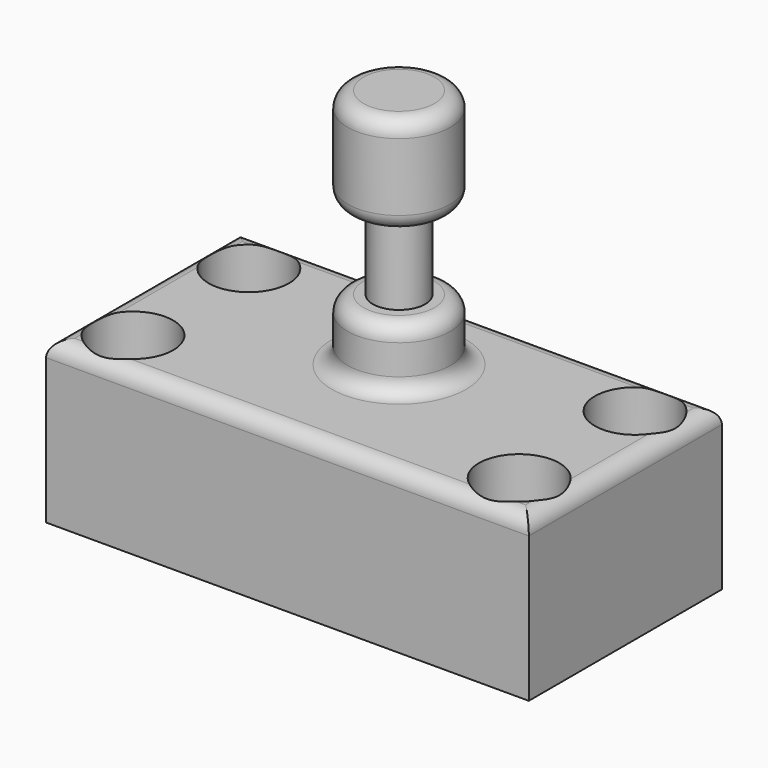
from build123d import *

# Parameters (mm, degrees)
F0_W        = 76.2
F0_H        = 38.1
F1_DEPTH    = 25.4
F2_R        = 6.35
F3_DEPTH    = 25.4
F4_R        = 8.1070086834
F5_DEPTH    = 38.1
F6_W        = 12.6953125
F6_H        = 12.6953087747
F8_T3_DEPTH = 50.8048285845
F8_T5_DEPTH = 88.9048285845


# Not quite as in the source:
# - a fillet or chamfer that OpenCascade refuses, or shapes differently, is made with other operations: its cross-section is extruded or revolved along the edge and cut away or added


with BuildPart() as f1:
    # F0 (on Top) → F1 (new body)
    with BuildSketch(Plane.XY):
        with Locations((-0.0034216791, -2.9583363167)):
            Rectangle(F0_W, F0_H)
    extrude(amount=F1_DEPTH)

    # F2 (on Top) → F3 (cut)
    with BuildSketch(Plane.XY):
        with Locations((-30.4834216791, 8.4716636833)):
            Circle(F2_R)
        with Locations((30.4765783209, 8.4716636833)):
            Circle(F2_R)
        with Locations((-30.4834216791, -14.3883363167)):
            Circle(F2_R)
        with Locations((30.4765783209, -14.3883363167)):
            Circle(F2_R)
    extrude(amount=F3_DEPTH, mode=Mode.SUBTRACT)

    # F4 (on face) → F5 (join)
    with BuildSketch(Plane.XY.offset(25.4)):
        Circle(F4_R)
    extrude(amount=F5_DEPTH)

    # F6 (on Front) → F7 (revolve, cut)
    with BuildSketch(Plane.XZ):
        with Locations((-10.4810148478, 41.481198743)):
            Rectangle(F6_W, F6_H)
    revolve(axis=Axis((0, 0, 25.4), (0, 0, -1)), mode=Mode.SUBTRACT)

    # F8: fillet of radius 2.54 on 8 edges, made by hand

    # F8_s1 → F8_t2 (revolve)
    with BuildSketch(Plane.XZ):
        with BuildLine():
            ThreePointArc((10.6479743688, 25.3996), (8.8509574592, 26.1439487758), (8.1066086834, 27.9409656854))
            Line((8.1066086834, 27.9409656854), (7.8524721149, 27.9409656854))
            ThreePointArc((7.8524721149, 27.9409656854), (7.8528721149, 26.6704828427), (7.8528721149, 25.4))
            Line((7.8528721149, 25.4), (8.1070086834, 25.1458634315))
            ThreePointArc((8.1070086834, 25.1458634315), (9.3774915261, 25.1458634315), (10.6479743688, 25.1454634315))
            Line((10.6479743688, 25.1454634315), (10.6479743688, 25.3996))
        make_face()
    revolve(axis=Axis((0, 0, 25.4), (0, 0, 1)))

    # F8_s4 → F8_t3 (cut)
    with BuildSketch(Plane.XZ.offset(-22.4440779756)):
        with BuildLine():
            ThreePointArc((-38.1038216791, 22.8590343146), (-37.3594729034, 24.6560512242), (-35.5624559937, 25.4004))
            Line((-35.5624559937, 25.4004), (-35.5624559937, 25.6545365685))
            ThreePointArc((-35.5624559937, 25.6545365685), (-36.8329388364, 25.6541365685), (-38.1034216791, 25.6541365685))
            Line((-38.1034216791, 25.6541365685), (-38.3575582477, 25.4))
            ThreePointArc((-38.3575582477, 25.4), (-38.3575582477, 24.1295171573), (-38.3579582477, 22.8590343146))
            Line((-38.3579582477, 22.8590343146), (-38.1038216791, 22.8590343146))
        make_face()
        with BuildLine():
            ThreePointArc((38.0969783209, 22.8590343146), (37.3526295451, 24.6560512242), (35.5556126354, 25.4004))
            Line((35.5556126354, 25.4004), (35.5556126354, 25.6545365685))
            ThreePointArc((35.5556126354, 25.6545365685), (36.8260954781, 25.6541365685), (38.0965783209, 25.6541365685))
            Line((38.0965783209, 25.6541365685), (38.3507148894, 25.4))
            ThreePointArc((38.3507148894, 25.4), (38.3507148894, 24.1295171573), (38.3511148894, 22.8590343146))
            Line((38.3511148894, 22.8590343146), (38.0969783209, 22.8590343146))
        make_face()
    extrude(amount=F8_T3_DEPTH, mode=Mode.SUBTRACT)

    # F8_s6 → F8_t5 (cut)
    with BuildSketch(Plane.YZ.offset(-44.4558359714)):
        with BuildLine():
            ThreePointArc((-19.4673706312, 25.4004), (-21.2643875409, 24.6560512242), (-22.0087363167, 22.8590343146))
            Line((-22.0087363167, 22.8590343146), (-22.2628728852, 22.8590343146))
            ThreePointArc((-22.2628728852, 22.8590343146), (-22.2624728852, 24.1295171573), (-22.2624728852, 25.4))
            Line((-22.2624728852, 25.4), (-22.0083363167, 25.6541365685))
            ThreePointArc((-22.0083363167, 25.6541365685), (-20.7378534739, 25.6541365685), (-19.4673706312, 25.6545365685))
            Line((-19.4673706312, 25.6545365685), (-19.4673706312, 25.4004))
        make_face()
        with BuildLine():
            ThreePointArc((16.0920636833, 22.8590343146), (15.3477149076, 24.6560512242), (13.5506979979, 25.4004))
            Line((13.5506979979, 25.4004), (13.5506979979, 25.6545365685))
            ThreePointArc((13.5506979979, 25.6545365685), (14.8211808406, 25.6541365685), (16.0916636833, 25.6541365685))
            Line((16.0916636833, 25.6541365685), (16.3458002519, 25.4))
            ThreePointArc((16.3458002519, 25.4), (16.3458002519, 24.1295171573), (16.3462002519, 22.8590343146))
            Line((16.3462002519, 22.8590343146), (16.0920636833, 22.8590343146))
        make_face()
    extrude(amount=F8_T5_DEPTH, mode=Mode.SUBTRACT)

    # F8_s7 → F8_t8 (revolve, cut)
    with BuildSketch(Plane.XZ):
        with BuildLine():
            ThreePointArc((8.1074086834, 32.5925786702), (7.3630599076, 34.3895955798), (5.566042998, 35.1339443556))
            Line((5.566042998, 35.1339443556), (5.566042998, 35.3880809242))
            ThreePointArc((5.566042998, 35.3880809242), (6.8365258407, 35.3876809242), (8.1070086834, 35.3876809242))
            Line((8.1070086834, 35.3876809242), (8.361145252, 35.1335443556))
            ThreePointArc((8.361145252, 35.1335443556), (8.361145252, 33.8630615129), (8.361545252, 32.5925786702))
            Line((8.361545252, 32.5925786702), (8.1074086834, 32.5925786702))
        make_face()
    revolve(axis=Axis((0, 0, 35.1335443556), (0, 0, -1)), mode=Mode.SUBTRACT)

    # F8_s9 → F8_t10 (revolve, cut)
    with BuildSketch(Plane.XZ):
        with BuildLine():
            ThreePointArc((5.566042998, 47.8284531303), (7.3630599076, 48.5728019061), (8.1074086834, 50.3698188158))
            Line((8.1074086834, 50.3698188158), (8.361545252, 50.3698188158))
            ThreePointArc((8.361545252, 50.3698188158), (8.361145252, 49.0993359731), (8.361145252, 47.8288531303))
            Line((8.361145252, 47.8288531303), (8.1070086834, 47.5747165618))
            ThreePointArc((8.1070086834, 47.5747165618), (6.8365258407, 47.5747165618), (5.566042998, 47.5743165618))
            Line((5.566042998, 47.5743165618), (5.566042998, 47.8284531303))
        make_face()
    revolve(axis=Axis((0, 0, 47.8288531303), (0, 0, -1)), mode=Mode.SUBTRACT)

    # F8_s11 → F8_t12 (revolve, cut)
    with BuildSketch(Plane.XZ):
        with BuildLine():
            ThreePointArc((8.1074086834, 60.9590343146), (7.3630599076, 62.7560512242), (5.566042998, 63.5004))
            Line((5.566042998, 63.5004), (5.566042998, 63.7545365685))
            ThreePointArc((5.566042998, 63.7545365685), (6.8365258407, 63.7541365685), (8.1070086834, 63.7541365685))
            Line((8.1070086834, 63.7541365685), (8.361145252, 63.5))
            ThreePointArc((8.361145252, 63.5), (8.361145252, 62.2295171573), (8.361545252, 60.9590343146))
            Line((8.361545252, 60.9590343146), (8.1074086834, 60.9590343146))
        make_face()
    revolve(axis=Axis((0, 0, 63.5), (0, 0, 1)), mode=Mode.SUBTRACT)


solid = f1.part
